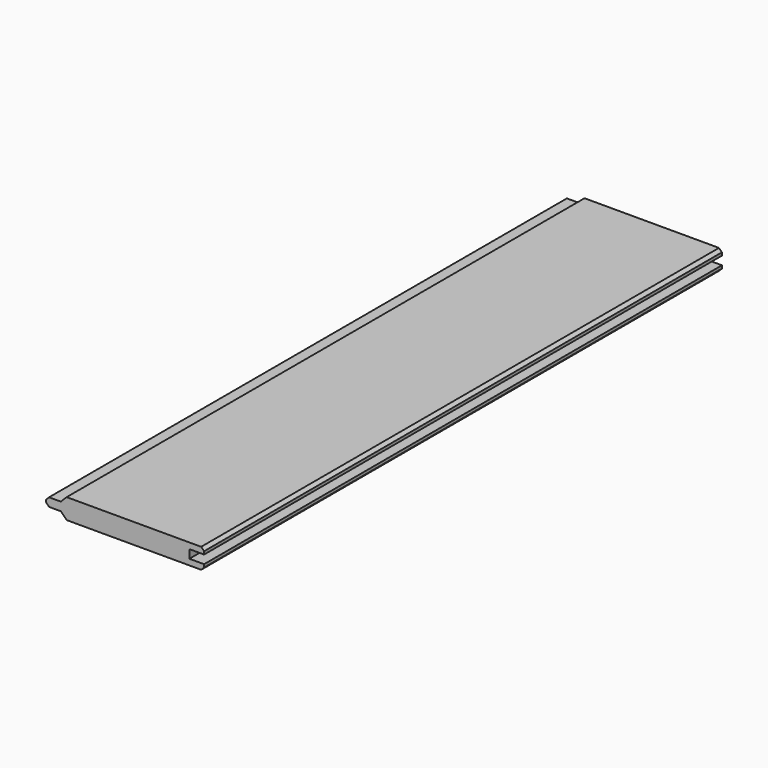
from build123d import *

# Parameters (mm, degrees)
F1_DEPTH = 558.8
F2_SIZE  = 2.54
F3_SIZE  = 5.07999


# Not quite as in the source:
# - a fillet or chamfer is up to 0.001 mm smaller than in the source, because OpenCascade refuses the exact size


with BuildPart() as f1:
    # F0 (on Front) → F1 (new body)
    with BuildSketch(Plane.XZ):
        Polygon((68.199, 3.6576), (68.199, 8.7376), (-55.499, 8.7376), (-55.499, 3.6576), (-68.199, 3.6576), (-68.199, -3.6576), (-55.499, -3.6576), (-55.499, -8.7376), (68.199, -8.7376), (68.199, -3.6576), (55.499, -3.6576), (55.499, 3.6576), align=None)
    extrude(amount=F1_DEPTH)

    # F2
    f2_edges = [f1.edges().sort_by_distance(p)[0] for p in [
        (68.199, -279.4, 8.7376),
        (68.199, -279.4, -8.7376),
        (-68.199, -279.4, 3.6576),
        (-68.199, -279.4, -3.6576),
    ]]
    chamfer(f2_edges, length=F2_SIZE)

    # F3 (size 5.08 in the source; OpenCascade refuses exactly that, so slightly less here)
    f3_edges = [f1.edges().sort_by_distance(p)[0] for p in [
        (-55.499, -279.4, 8.7376),
        (-55.499, -279.4, -8.7376),
    ]]
    chamfer(f3_edges, length=F3_SIZE)


solid = f1.part
